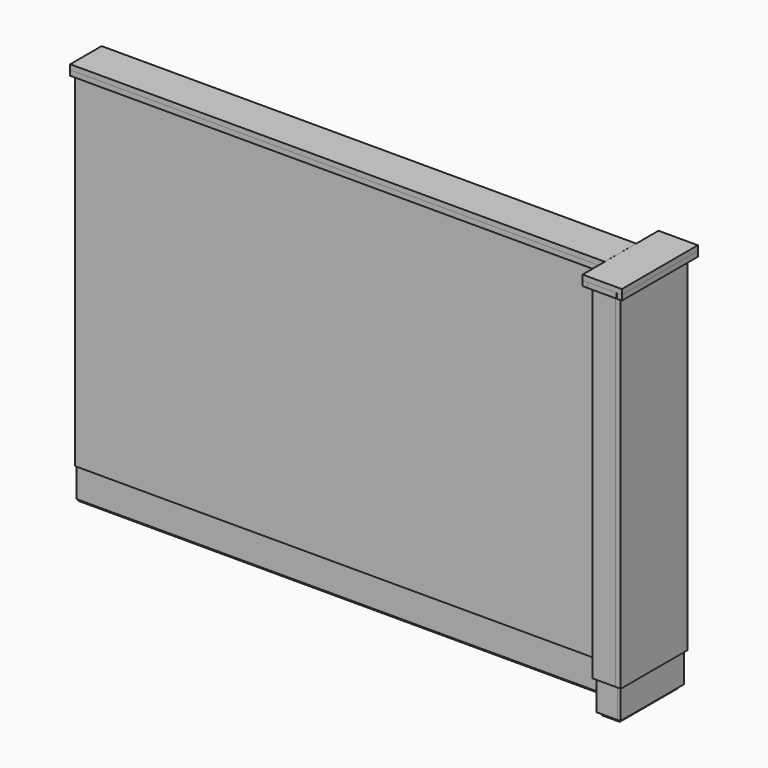
from build123d import *

# Parameters (mm, degrees)
F0_W      = 60
F0_H      = 30
F0_W_2    = 52
F0_H_2    = 22
F1_DEPTH  = 1823
F2_W      = 30
F2_H      = 60
F2_W_2    = 22
F2_H_2    = 52
F3_DEPTH  = 1223
F4_W      = 60
F4_H      = 30
F4_W_2    = 52
F4_H_2    = 22
F5_DEPTH  = 123
F6_W      = 60
F6_H      = 30
F6_W_2    = 52
F6_H_2    = 22
F6_W_3    = 30
F6_H_3    = 60
F6_W_4    = 22
F6_H_4    = 52
F7_DEPTH  = 1223
F9_W      = 1820.4
F9_H      = 1171.7
F10_DEPTH = 17
F11_W     = 1820.4
F11_H     = 100
F12_DEPTH = 10
F16_DEPTH = 1171.7
F18_DEPTH = 100
F19_W     = 17
F19_H     = 73.4
F20_DEPTH = 1173
F21_W     = 10
F21_H     = 7
F21_H_2   = 73.4
F22_DEPTH = 100
F21_H_3   = 80.4
F23_W     = 1787.13
F23_H     = 131.4
F24_DEPTH = 17
F25_W     = 35.7
F25_H     = 60
F26_DEPTH = 17
F28_DEPTH = 17
F30_R     = 15
F31_DEPTH = 10
F32_R     = 7
F33_DEPTH = 30.001
F34_R     = 7
F35_DEPTH = 60
F36_R     = 15
F37_DEPTH = 10
F39_W     = 0.1
F39_H     = 282
F40_DEPTH = 1283.001
F41_W     = 0.1
F41_H     = 337.4
F41_H_2   = 163.9194041491
F41_H_3   = 431.6920638084
F42_DEPTH = 1283.001


# Not quite as in the source:
# - a feature of the source that left no trace in its solid (it failed there, or was rolled back) is left out


with BuildPart() as f1:
    # F0 (on Right) → F1 (new body)
    with BuildSketch(Plane.YZ):
        with Locations((0, 15)):
            Rectangle(F0_W, F0_H)
        with Locations((0, 15)):
            Rectangle(F0_W_2, F0_H_2, mode=Mode.SUBTRACT)
    extrude(amount=F1_DEPTH)



with BuildPart() as f1b:
    # F0 (on Right) → F1, piece 2 (new body)
    with BuildSketch(Plane.YZ):
        with Locations((0, 1268)):
            Rectangle(F0_W, F0_H)
        with Locations((0, 1268)):
            Rectangle(F0_W_2, F0_H_2, mode=Mode.SUBTRACT)
    extrude(amount=F1_DEPTH)


with BuildPart() as f1_1:
    add(f1.part)

    add(f1b.part)  # F3 merges F1b
    # F2 (on face) → F3 (join, through all)
    with BuildSketch(Plane.XY.offset(30)):
        with Locations((15, 0)):
            Rectangle(F2_W, F2_H)
        with Locations((15, 0)):
            Rectangle(F2_W_2, F2_H_2, mode=Mode.SUBTRACT)
    extrude(amount=F3_DEPTH)

    # F4 (on Front) → F5 (join, symmetric)
    with BuildSketch(Plane.XZ):
        with Locations((1853, 1268)):
            Rectangle(F4_W, F4_H)
        with Locations((1853, 1268)):
            Rectangle(F4_W_2, F4_H_2, mode=Mode.SUBTRACT)
        with Locations((1853, 15)):
            Rectangle(F4_W, F4_H)
        with Locations((1853, 15)):
            Rectangle(F4_W_2, F4_H_2, mode=Mode.SUBTRACT)
    extrude(amount=F5_DEPTH, both=True)

    # F6 (on face) → F7 (join, through all)
    with BuildSketch(Plane.XY.offset(30)):
        with Locations((1853, 108)):
            Rectangle(F6_W, F6_H)
        with Locations((1853, 108)):
            Rectangle(F6_W_2, F6_H_2, mode=Mode.SUBTRACT)
        with Locations((1853, -108)):
            Rectangle(F6_W, F6_H)
        with Locations((1853, -108)):
            Rectangle(F6_W_2, F6_H_2, mode=Mode.SUBTRACT)
        with Locations((1868, 0)):
            Rectangle(F6_W_3, F6_H_3)
        with Locations((1868, 0)):
            Rectangle(F6_W_4, F6_H_4, mode=Mode.SUBTRACT)
        with Locations((1250.3333333333, 0)):
            Rectangle(F6_W_3, F6_H_3)
        with Locations((1250.3333333333, 0)):
            Rectangle(F6_W_4, F6_H_4, mode=Mode.SUBTRACT)
        with Locations((632.6666666667, 0)):
            Rectangle(F6_W_3, F6_H_3)
        with Locations((632.6666666667, 0)):
            Rectangle(F6_W_4, F6_H_4, mode=Mode.SUBTRACT)
    extrude(amount=F7_DEPTH)

    # F29: union 

    # F30 (on face) → F31 (cut)
    with BuildSketch(Plane.XY.offset(30)):
        with Locations((1853, 63)):
            Circle(F30_R)
        with Locations((1853, -63)):
            Circle(F30_R)
        with Locations((180, 0)):
            Circle(F30_R)
        with Locations((467.6666666667, 0)):
            Circle(F30_R)
        with Locations((797.6666666667, 0)):
            Circle(F30_R)
        with Locations((1085.3333333333, 0)):
            Circle(F30_R)
        with Locations((1415.3333333333, 0)):
            Circle(F30_R)
        with Locations((1673, 0)):
            Circle(F30_R)
    extrude(amount=-F31_DEPTH, mode=Mode.SUBTRACT)

    # F32 (on face) → F33 (cut, through all)
    with BuildSketch(Plane.XY.offset(30)):
        with Locations((180, 0)):
            Circle(F32_R)
        with Locations((467.6666666667, 0)):
            Circle(F32_R)
        with Locations((797.6666666667, 0)):
            Circle(F32_R)
        with Locations((1085.3333333333, 0)):
            Circle(F32_R)
        with Locations((1415.3333333333, 0)):
            Circle(F32_R)
        with Locations((1673, 0)):
            Circle(F32_R)
        with Locations((1853, 63)):
            Circle(F32_R)
        with Locations((1853, -63)):
            Circle(F32_R)
    extrude(amount=-F33_DEPTH, mode=Mode.SUBTRACT)

    # F34 (on face) → F35 (cut)
    with BuildSketch(Plane(origin=(0, 0, 0), x_dir=(0, -1, 0), z_dir=(-1, 0, 0))):
        with Locations((0, 126)):
            Circle(F34_R)
        with Locations((0, 446)):
            Circle(F34_R)
        with Locations((0, 766)):
            Circle(F34_R)
        with Locations((0, 1086)):
            Circle(F34_R)
        with Locations((0, 1406)):
            Circle(F34_R)
    extrude(amount=-F35_DEPTH, mode=Mode.SUBTRACT)

    # F36 (on face) → F37 (cut)
    with BuildSketch(Plane.YZ.offset(30)):
        with Locations((0, 126)):
            Circle(F36_R)
        with Locations((0, 1086)):
            Circle(F36_R)
        with Locations((0, 766)):
            Circle(F36_R)
        with Locations((0, 446)):
            Circle(F36_R)
    extrude(amount=-F37_DEPTH, mode=Mode.SUBTRACT)


with BuildPart() as f10:
    # F9 (on offset) → F10 (new body)
    with BuildSketch(Plane.XZ.offset(30)):
        with Locations((911.5, 695.85)):
            Rectangle(F9_W, F9_H)
    extrude(amount=F10_DEPTH)


with BuildPart() as f12:
    # F11 (on offset) → F12 (new body)
    with BuildSketch(Plane.XZ.offset(30)):
        with Locations((911.5, 60)):
            Rectangle(F11_W, F11_H)
    extrude(amount=F12_DEPTH)


with BuildPart() as f13_1:
    # F13: instance of F10
    add(f10.part.mirror(Plane.XZ))


with BuildPart() as f13_2:
    # F13: instance of F12
    add(f12.part.mirror(Plane.XZ))


with BuildPart() as f16:
    # F15 (on offset) → F16 (new body, through all)
    with BuildSketch(Plane.XY.offset(1281.7)):
        Polygon((1900, -140), (1900, 140), (1883, 140), (1806, 140), (1806, 123), (1883, 123), (1883, -123), (1806, -123), (1806, -140), (1883, -140), align=None)
    extrude(amount=-F16_DEPTH)


with BuildPart() as f18:
    # F17 (on face) → F18 (new body, through all)
    with BuildSketch(Plane(origin=(0, 0, 110), x_dir=(1, 0, 0), z_dir=(0, 0, -1))):
        Polygon((1883, -123), (1813, -123), (1813, -133), (1893, -133), (1893, 133), (1813, 133), (1813, 123), (1883, 123), align=None)
    extrude(amount=F18_DEPTH)


with BuildPart() as f20:
    # F19 (on face) → F20 (new body, through all)
    with BuildSketch(Plane.XY.offset(1283)):
        with Locations((1814.5, -85)):
            Rectangle(F19_W, F19_H)
    extrude(amount=-F20_DEPTH)


with BuildPart() as f20b:
    # F19 (on face) → F20, piece 2 (new body, through all)
    with BuildSketch(Plane.XY.offset(1283)):
        with Locations((1814.5, 85)):
            Rectangle(F19_W, F19_H)
    extrude(amount=-F20_DEPTH)


with BuildPart() as f22:
    # F21 (on face) → F22 (new body, through all)
    with BuildSketch(Plane(origin=(0, 0, 110), x_dir=(1, 0, 0), z_dir=(0, 0, -1))):
        with Locations((1818, -44.8)):
            Rectangle(F21_W, F21_H)
        with Locations((1818, -85)):
            Rectangle(F21_W, F21_H_2)
    extrude(amount=F22_DEPTH)


with BuildPart() as f22b:
    # F21 (on face) → F22, piece 2 (new body, through all)
    with BuildSketch(Plane(origin=(0, 0, 110), x_dir=(1, 0, 0), z_dir=(0, 0, -1))):
        with Locations((1818, 81.5)):
            Rectangle(F21_W, F21_H_3)
    extrude(amount=F22_DEPTH)


with BuildPart() as f24:
    # F23 (on face) → F24 (new body)
    with BuildSketch(Plane.XY.offset(1283)):
        with Locations((893.565, 0)):
            Rectangle(F23_W, F23_H)
    extrude(amount=F24_DEPTH)


with BuildPart() as f26:
    # F25 (on face) → F26 (new body)
    with BuildSketch(Plane.XY.offset(1283)):
        Polygon((1918.7, 158.7), (1787.3, 158.7), (1787.3, 30), (1823, 30), (1823, 123), (1883, 123), (1883, -123), (1823, -123), (1823, -30), (1787.3, -30), (1787.3, -158.7), (1918.7, -158.7), align=None)
        with Locations((1805.15, 0)):
            Rectangle(F25_W, F25_H)
        Polygon((1823, 123), (1823, 30), (1823, -30), (1823, -123), (1883, -123), (1883, 123), align=None)
    extrude(amount=F26_DEPTH)


with BuildPart() as f28:
    # F27 (on face) → F28 (new body)
    with BuildSketch(Plane(origin=(0, 0, 1283), x_dir=(1, 0, 0), z_dir=(0, 0, -1))):
        Polygon((0, -48.7), (0, -65.7), (1787.3, -65.7), (1804.3, -65.7), (1804.3, -48.7), align=None)
        Polygon((1804.3, -65.7), (1787.3, -65.7), (1787.3, -158.7), (1804.3, -158.7), (1804.3, -141.7), align=None)
        Polygon((1901.7, -141.7), (1804.3, -141.7), (1804.3, -158.7), (1918.7, -158.7), (1918.7, -141.7), (1918.7, 141.7), (1918.7, 158.7), (1804.3, 158.7), (1804.3, 141.7), (1901.7, 141.7), align=None)
        Polygon((1804.3, 65.7), (1804.3, 141.7), (1804.3, 158.7), (1787.3, 158.7), (1787.3, 65.7), align=None)
        Polygon((1804.3, 48.7), (1804.3, 65.7), (1787.3, 65.7), (0, 65.7), (0, 48.7), align=None)
    extrude(amount=F28_DEPTH)

    # F41 (on offset) → F42 (cut, through all)
    with BuildSketch(Plane.XY.offset(1283)):
        with Locations((1901.65, 0)):
            Rectangle(F41_W, F41_H)
        with Locations((1787.25, 3.0303150415)):
            Rectangle(F41_W, F41_H_2)
        with Locations((1804.25, 10.9124034643)):
            Rectangle(F41_W, F41_H_3)
    extrude(amount=-F42_DEPTH, mode=Mode.SUBTRACT)


with BuildPart() as f40_tool:
    # F39 (on offset) → F40 (new body, through all)
    with BuildSketch(Plane.XY.offset(1283)):
        with Locations((1882.95, 0)):
            Rectangle(F39_W, F39_H)
    extrude(amount=-F40_DEPTH)


with BuildPart() as f16_1:
    add(f16.part)

    # F40: cut by f40_tool
    add(f40_tool.part, mode=Mode.SUBTRACT)


with BuildPart() as f18_1:
    add(f18.part)

    # F40: cut by f40_tool
    add(f40_tool.part, mode=Mode.SUBTRACT)


solid = Compound([f1_1.part, f10.part, f12.part, f13_1.part, f13_2.part, f20.part, f20b.part, f22.part, f22b.part, f24.part, f26.part, f28.part, f16_1.part, f18_1.part])
